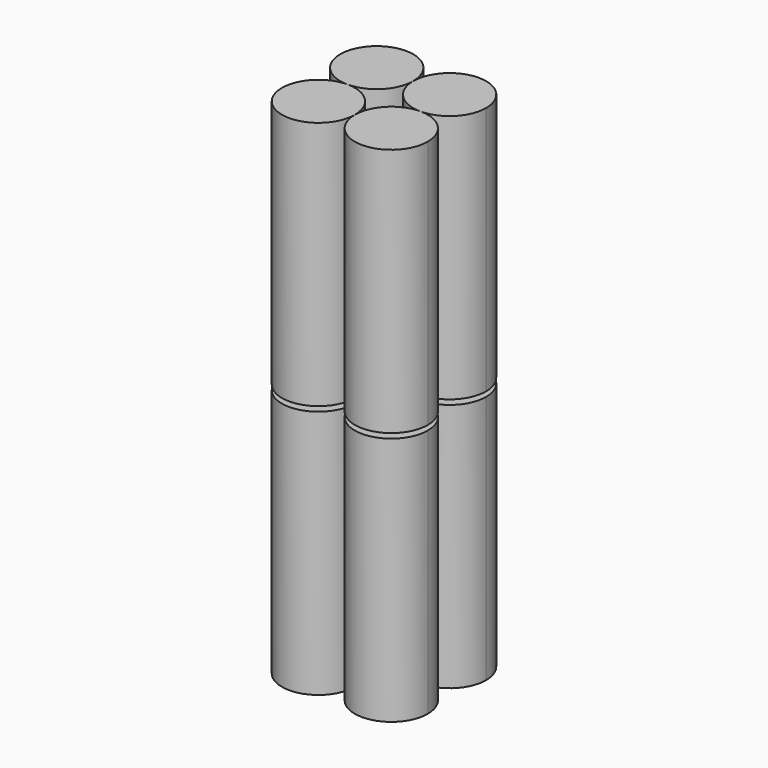
from build123d import *

# Parameters (mm, degrees)
F1_DEPTH = 65
F4_DEPTH = 65


with BuildPart() as f1:
    # F0 (on Top) → F1 (new body)
    with BuildSketch(Plane.XY):
        with BuildLine():
            ThreePointArc((19, 9.5), (9.5, 19), (0, 9.5))
            ThreePointArc((0, 9.5), (2.7824855787, 2.7824855787), (9.5, 0))
            ThreePointArc((9.5, 0), (16.2175144213, 2.7824855787), (19, 9.5))
        make_face()
    extrude(amount=F1_DEPTH)


with BuildPart() as f1b:
    # F0 (on Top) → F1, piece 2 (new body)
    with BuildSketch(Plane.XY):
        with BuildLine():
            ThreePointArc((19, -9.5), (16.2175144213, -2.7824855787), (9.5, 0))
            ThreePointArc((9.5, 0), (2.7824855787, -2.7824855787), (0, -9.5))
            ThreePointArc((0, -9.5), (9.5, -19), (19, -9.5))
        make_face()
    extrude(amount=F1_DEPTH)


with BuildPart() as f1c:
    # F0 (on Top) → F1, piece 3 (new body)
    with BuildSketch(Plane.XY):
        with BuildLine():
            ThreePointArc((0, -9.5), (-2.7824855787, -2.7824855787), (-9.5, 0))
            ThreePointArc((-9.5, 0), (-16.2175144213, -16.2175144213), (0, -9.5))
        make_face()
    extrude(amount=F1_DEPTH)


with BuildPart() as f1d:
    # F0 (on Top) → F1, piece 4 (new body)
    with BuildSketch(Plane.XY):
        with BuildLine():
            ThreePointArc((-9.5, 0), (-2.7824855787, 2.7824855787), (0, 9.5))
            ThreePointArc((0, 9.5), (-16.2175144213, 16.2175144213), (-9.5, 0))
        make_face()
    extrude(amount=F1_DEPTH)


with BuildPart() as f4:
    # F3 (on offset) → F4 (new body)
    with BuildSketch(Plane.XY.offset(66.27)):
        with BuildLine():
            ThreePointArc((0, 9.5), (2.7824856048, 2.7824855527), (9.5000000736, 0))
            ThreePointArc((9.5000000736, 0), (16.2175144473, 2.7824856048), (19, 9.5))
            ThreePointArc((19, 9.5), (9.5, 19), (0, 9.5))
        make_face()
    extrude(amount=F4_DEPTH)


with BuildPart() as f4b:
    # F3 (on offset) → F4, piece 2 (new body)
    with BuildSketch(Plane.XY.offset(66.27)):
        with BuildLine():
            ThreePointArc((9.5000000736, 0), (2.7824856048, -2.7824855527), (0, -9.5))
            ThreePointArc((0, -9.5), (9.5, -19), (19, -9.5))
            ThreePointArc((19, -9.5), (16.2175144473, -2.7824856048), (9.5000000736, 0))
        make_face()
    extrude(amount=F4_DEPTH)


with BuildPart() as f4c:
    # F3 (on offset) → F4, piece 3 (new body)
    with BuildSketch(Plane.XY.offset(66.27)):
        with BuildLine():
            ThreePointArc((-9.4999999957, 0), (-16.2175144228, -16.2175144197), (0, -9.5))
            ThreePointArc((0, -9.5), (-2.7824855772, -2.7824855803), (-9.4999999957, 0))
        make_face()
    extrude(amount=F4_DEPTH)


with BuildPart() as f4d:
    # F3 (on offset) → F4, piece 4 (new body)
    with BuildSketch(Plane.XY.offset(66.27)):
        with BuildLine():
            ThreePointArc((0, 9.5), (-16.2175144228, 16.2175144197), (-9.4999999957, 0))
            ThreePointArc((-9.4999999957, 0), (-2.7824855772, 2.7824855803), (0, 9.5))
        make_face()
    extrude(amount=F4_DEPTH)


solid = Compound([f1.part, f1b.part, f1c.part, f1d.part, f4.part, f4b.part, f4c.part, f4d.part])
